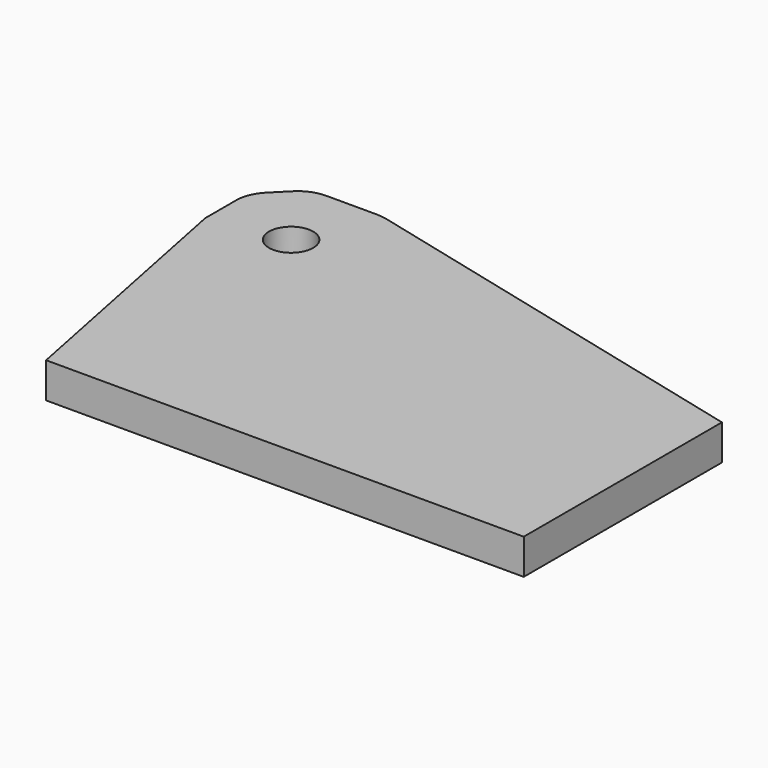
from build123d import *

# Parameters (mm, degrees)
F0_R        = 6.25
F1_DEPTH    = 10
F2_T1_DEPTH = 18.1439634323
F2_T3_DEPTH = 61.4336597593
F3_R        = 10


# Not quite as in the source:
# - a fillet or chamfer that OpenCascade refuses, or shapes differently, is made with other operations: its cross-section is extruded or revolved along the edge and cut away or added
# - two fillets or chamfers of one size are made in one step


with BuildPart() as f1:
    # F0 (on Top) → F1 (new body)
    with BuildSketch(Plane.XY):
        Polygon((0, 73.75), (15, -1.25), (150, -1.25), (150, 68.75), (30, 98.75), (0, 98.75), align=None)
        with Locations((21.25, 77.5)):
            Circle(F0_R, mode=Mode.SUBTRACT)
    extrude(amount=F1_DEPTH)

    # F2: chamfer of 10 on 2 edges, made by hand

    # F2_s2 → F2_t1 (cut)
    with BuildSketch(Plane.XY.offset(-4.0719817161)):
        Polygon((31.1942999942, 98.4514250015), (28.7689437438, 98.75), (30, 98.75), align=None)
    extrude(amount=F2_T1_DEPTH, mode=Mode.SUBTRACT)

    # F2_s4 → F2_t3 (cut)
    with BuildSketch(Plane.XY.offset(-25.7168298797)):
        Polygon((10, 98.75), (0, 88.75), (0, 98.75), align=None)
    extrude(amount=F2_T3_DEPTH, mode=Mode.SUBTRACT)

    # F3
    f3_edges = [f1.edges().sort_by_distance(p)[0] for p in [
        (0, 88.75, 5),
        (10, 98.75, 5),
        (28.768944, 98.75, 5),
    ]]
    fillet(f3_edges, radius=F3_R)


solid = f1.part
